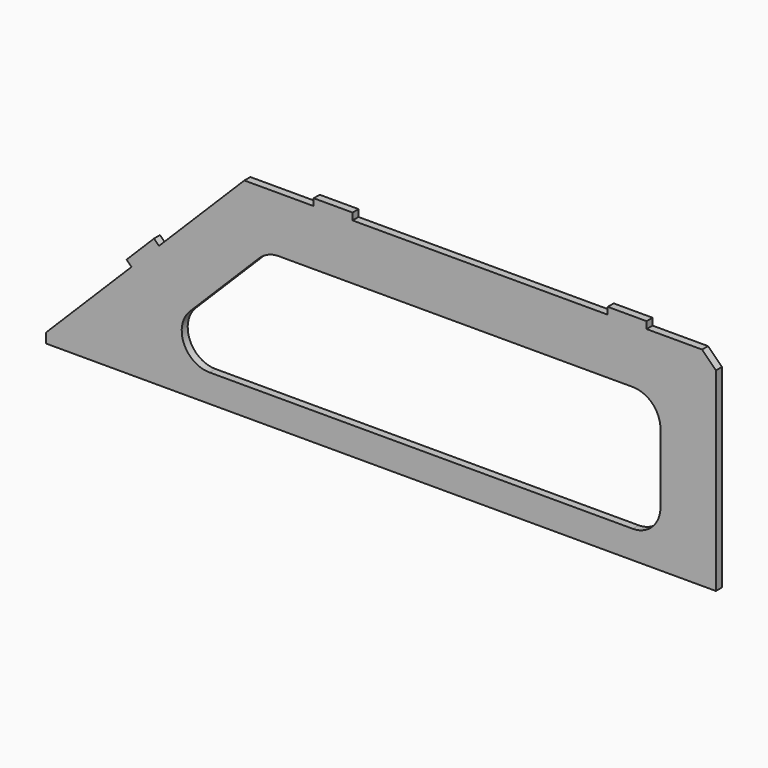
from build123d import *

# Parameters (mm, degrees)
F1_DEPTH = 3.429


# Not quite as in the source:
# - ends of sketch curves that miss each other by under 0.0002 mm in the source are joined


with BuildPart() as f1:
    # F0 (on Front) → F1 (new body)
    with BuildSketch(Plane.XZ):
        Polygon((718.4461374, -491.0265008), (700.6661374, -491.0265008), (700.6661374, -494.2015008), (668.9161374, -494.2015008), (629.8223878, -533.2952504), (627.5773072, -531.0501952), (615.0049422, -543.6225348), (617.2500228, -545.8676154), (578.1562732, -584.961365), (578.1562732, -589.4515008), (884.8161374, -589.4515008), (884.8161374, -500.5515008), (878.4661374, -494.2015008), (853.0661374, -494.2015008), (853.0661374, -491.0265008), (835.2861374, -491.0265008), (835.2861374, -494.2015008), (718.4461374, -494.2015008), align=None)
        with BuildLine():
            ThreePointArc((859.4161374, -564.0515008), (855.6963935211, -573.0317569211), (846.7161374, -576.7515008))
            Line((846.7161374, -576.7515008), (652.9476654, -576.7515008))
            ThreePointArc((652.9476654, -576.7515008), (641.2143919005, -568.9115720944), (643.9674219789, -555.0712319789))
            Line((643.9674219789, -555.0712319789), (675.7174192, -523.3212292))
            ThreePointArc((675.7174192, -523.3212292), (679.8375941056, -520.5682273005), (684.6976654, -519.6015008))
            Line((684.6976654, -519.6015008), (846.7161374, -519.6015008))
            ThreePointArc((846.7161374, -519.6015008), (855.6963935211, -523.3212446789), (859.4161374, -532.3015008))
            Line((859.4161374, -532.3015008), (859.4161374, -564.0515008))
        make_face(mode=Mode.SUBTRACT)
    extrude(amount=F1_DEPTH)


solid = f1.part
